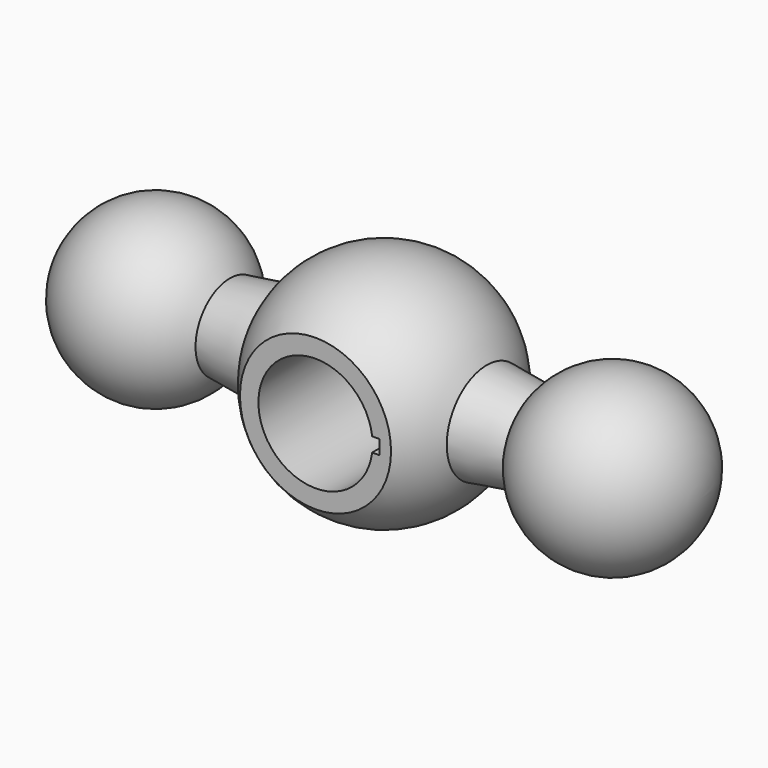
from build123d import *
from build123d import SkipClean  # not in build123d's __all__

# Parameters (mm, degrees)
F8_W          = 16.8005208253
F8_H          = 3.175
F1_DEPTH      = 12.701
F1_DEPTH_BACK = 12.701
F3_DEPTH      = 19.05
F5_R          = 3.175
F6_DEPTH      = 13.255625


with BuildPart() as f7:
    # F0 (on Top) → F7 (revolve)
    with BuildSketch(Plane.XY):
        with BuildLine():
            Line((17.151108029, 4.7625), (11.4200738149, 5.55625))
            ThreePointArc((11.4200738149, 5.55625), (0, 12.7), (-11.4200738149, 5.55625))
            Line((-11.4200738149, 5.55625), (-17.151108029, 4.7625))
            ThreePointArc((-17.151108029, 4.7625), (-27.8652514046, 9.2004434954), (-34.925, 0))
            Line((-34.925, 0), (34.925, 0))
            ThreePointArc((34.925, 0), (27.8652514046, 9.2004434954), (17.151108029, 4.7625))
        make_face()
    revolve(axis=Axis((0, 0, 0), (1, 0, 0)))

    # F8 (on Top) → F1 (cut, two sides)
    with BuildSketch(Plane.XY) as f1_sk:
        with Locations((0, 11.1125)):
            Rectangle(F8_W, F8_H)
        with Locations((0, -11.1125)):
            Rectangle(F8_W, F8_H)
    with SkipClean():  # cleaning this boolean's faces spoils the solid; the shape is the same uncleaned
        extrude(amount=F1_DEPTH, mode=Mode.SUBTRACT)
        extrude(f1_sk.sketch, amount=-F1_DEPTH_BACK, mode=Mode.SUBTRACT)

    # F2 (on face) → F3 (cut, through all)
    with BuildSketch(Plane.XZ.offset(9.525)):
        with BuildLine():
            ThreePointArc((6.3001953095, -0.79375), (6.3375365962, -0.3976554946), (6.35, 0))
            ThreePointArc((6.35, 0), (6.3375365962, 0.3976554946), (6.3001953095, 0.79375))
            ThreePointArc((6.3001953095, 0.79375), (-6.35, 0), (6.3001953095, -0.79375))
        make_face()
        with BuildLine():
            ThreePointArc((6.3001953095, 0.79375), (6.3375365962, 0.3976554946), (6.35, 0))
            ThreePointArc((6.35, 0), (6.3375365962, -0.3976554946), (6.3001953095, -0.79375))
            Line((6.3001953095, -0.79375), (7.14375, -0.79375))
            Line((7.14375, -0.79375), (7.14375, 0.79375))
            Line((7.14375, 0.79375), (6.3001953095, 0.79375))
        make_face()
    with SkipClean():  # cleaning this boolean's faces spoils the solid; the shape is the same uncleaned
        extrude(amount=-F3_DEPTH, mode=Mode.SUBTRACT)

    # F5 (on plane+point) → F6 (cut)
    with BuildSketch(Plane.XZ.offset(-9.525)):
        with Locations((25.4, 0)):
            Circle(F5_R)
        with Locations((-25.4, 0)):
            Circle(F5_R)
    extrude(amount=F6_DEPTH, mode=Mode.SUBTRACT)


solid = f7.part
